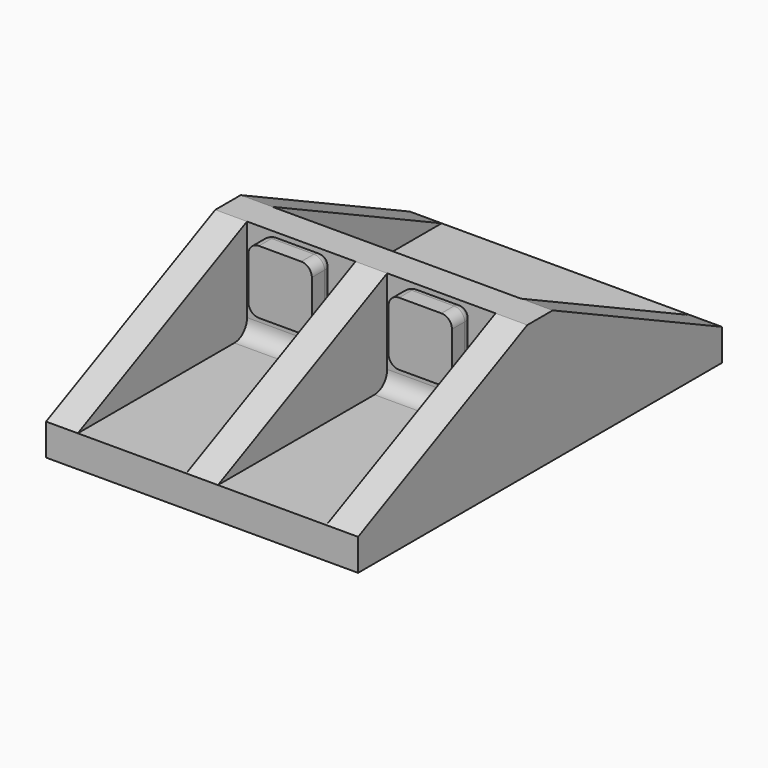
from build123d import *

# Parameters (mm, degrees)
F0_W             = 59
F0_H             = 86
F1_DEPTH         = 6
F3_DEPTH         = 19
F5_DEPTH         = 59.001
F7_R             = 3
F6_W             = 12
F6_H             = 12
F8_DEPTH         = 5
F9_R             = 2
F10_T1_DEPTH     = 8
F10_S5_W         = 2
F10_S5_H         = 2
F10_T6_DEPTH     = 2
F10_S11_W        = 2
F10_S11_H        = 2
F10_T12_DEPTH    = 2
F10_S17_W        = 2
F10_S17_H        = 2
F10_T18_DEPTH    = 2
F10_S23_W        = 2
F10_S23_H        = 2
F10_T24_DEPTH    = 2
F10_S1_T1_DEPTH  = 8
F10_S1_S5_W      = 2
F10_S1_S5_H      = 2
F10_S1_T6_DEPTH  = 2
F10_S1_S11_W     = 2
F10_S1_S11_H     = 2
F10_S1_T12_DEPTH = 2
F10_S1_S17_W     = 2
F10_S1_S17_H     = 2
F10_S1_T18_DEPTH = 2
F10_S1_S23_W     = 2
F10_S1_S23_H     = 2
F10_S1_T24_DEPTH = 2


# Not quite as in the source:
# - a fillet or chamfer that OpenCascade refuses, or shapes differently, is made with other operations: its cross-section is extruded or revolved along the edge and cut away or added


with BuildPart() as f1:
    # F0 (on Top) → F1 (new body)
    with BuildSketch(Plane.XY):
        Rectangle(F0_W, F0_H)
    extrude(amount=F1_DEPTH)

    # F2 (on face) → F3 (join)
    with BuildSketch(Plane.XY.offset(6)):
        Polygon((-23.5, 43), (-29.5, 43), (-29.5, -43), (-23.5, -43), (-23.5, -3), (-3, -3), (-3, -43), (3, -43), (3, -3), (23.5, -3), (23.5, -43), (29.5, -43), (29.5, 43), (23.5, 43), (23.5, 3), (-23.5, 3), align=None)
    extrude(amount=F3_DEPTH)

    # F4 (on face) → F5 (cut, through all)
    with BuildSketch(Plane.YZ.offset(29.5)):
        Polygon((-43, 25), (-43, 6), (-3, 25), align=None)
        Polygon((43, 25), (3, 25), (43, 6), align=None)
    extrude(amount=-F5_DEPTH, mode=Mode.SUBTRACT)

    # F7
    f7_edges = [f1.edges().sort_by_distance(p)[0] for p in [
        (-13.25, -3, 6),
        (13.25, -3, 6),
        (0, 3, 6),
    ]]
    fillet(f7_edges, radius=F7_R)


with BuildPart() as f8:
    # F6 (on face) → F8 (new body)
    with BuildSketch(Plane.XZ.offset(3)):
        with Locations((-13.25, 19)):
            Rectangle(F6_W, F6_H)
        with Locations((13.25, 19)):
            Rectangle(F6_W, F6_H)
    extrude(amount=F8_DEPTH)

    # F9
    f9_edges = [f8.edges().sort_by_distance(p)[0] for p in [
        (-7.25, -3, 19),
        (-13.25, -3, 25),
        (-19.25, -3, 19),
        (-13.25, -3, 13),
        (13.25, -3, 13),
        (7.25, -3, 19),
        (19.25, -3, 19),
        (13.25, -3, 25),
    ]]
    fillet(f9_edges, radius=F9_R)

    # F10: fillet of radius 2 on 4 edges, made by hand

    # F10_s2 → F10_t1 (cut)
    with BuildSketch(Plane.XZ.offset(5)):
        with BuildLine():
            ThreePointArc((-7.25, 15), (-7.8357864376, 13.5857864376), (-9.25, 13))
            Line((-9.25, 13), (-7.25, 13))
            Line((-7.25, 13), (-7.25, 15))
        make_face()
        with BuildLine():
            ThreePointArc((-19.25, 15), (-18.6642135624, 13.5857864376), (-17.25, 13))
            Line((-17.25, 13), (-19.25, 13))
            Line((-19.25, 13), (-19.25, 15))
        make_face()
        with BuildLine():
            ThreePointArc((-9.25, 25), (-7.8357864376, 24.4142135624), (-7.25, 23))
            Line((-7.25, 23), (-7.25, 25))
            Line((-7.25, 25), (-9.25, 25))
        make_face()
        with BuildLine():
            ThreePointArc((-17.25, 25), (-18.6642135624, 24.4142135624), (-19.25, 23))
            Line((-19.25, 23), (-19.25, 25))
            Line((-19.25, 25), (-17.25, 25))
        make_face()
    extrude(amount=F10_T1_DEPTH, mode=Mode.SUBTRACT)


with BuildPart() as f10_tool4:
    # F10_s5 → F10_t6 (new body)
    with BuildSketch(Plane.XY.offset(23)):
        with Locations((-18.25, -4)):
            Rectangle(F10_S5_W, F10_S5_H)
    extrude(amount=F10_T6_DEPTH)

    # F10_s7 → F10_t8 (revolve, cut)
    with BuildSketch(Plane(origin=(-17.25, -5, 23), x_dir=(0.7071067812, -0.7071067812, 0), z_dir=(-0.7071067812, -0.7071067812, 0))):
        with BuildLine():
            ThreePointArc((0, -2), (2, 0), (0, 2))
            Line((0, 2), (0, -2))
        make_face()
    revolve(axis=Axis((-17.25, -5, 23), (0, 0, 1)), mode=Mode.SUBTRACT)


with BuildPart() as f8_1:
    add(f8.part)

    # F10_t3: cut F10_tool4
    add(f10_tool4.part, mode=Mode.SUBTRACT)


with BuildPart() as f10_tool10:
    # F10_s11 → F10_t12 (new body)
    with BuildSketch(Plane.XY.offset(23)):
        with Locations((-8.25, -4)):
            Rectangle(F10_S11_W, F10_S11_H)
    extrude(amount=F10_T12_DEPTH)

    # F10_s13 → F10_t14 (revolve, cut)
    with BuildSketch(Plane(origin=(-9.25, -5, 23), x_dir=(-0.7071067812, -0.7071067812, 0), z_dir=(-0.7071067812, 0.7071067812, 0))):
        with BuildLine():
            ThreePointArc((0, -2), (2, 0), (0, 2))
            Line((0, 2), (0, -2))
        make_face()
    revolve(axis=Axis((-9.25, -5, 23), (0, 0, 1)), mode=Mode.SUBTRACT)


with BuildPart() as f8_2:
    add(f8_1.part)

    # F10_t9: cut F10_tool10
    add(f10_tool10.part, mode=Mode.SUBTRACT)


with BuildPart() as f10_tool16:
    # F10_s17 → F10_t18 (new body)
    with BuildSketch(Plane.YZ.offset(-17.25)):
        with Locations((-4, 14)):
            Rectangle(F10_S17_W, F10_S17_H)
    extrude(amount=-F10_T18_DEPTH)

    # F10_s19 → F10_t20 (revolve, cut)
    with BuildSketch(Plane(origin=(-17.25, -5, 15), x_dir=(0, -0.7071067812, 0.7071067812), z_dir=(0, -0.7071067812, -0.7071067812))):
        with BuildLine():
            ThreePointArc((0, -2), (2, 0), (0, 2))
            Line((0, 2), (0, -2))
        make_face()
    revolve(axis=Axis((-17.25, -5, 15), (-1, 0, 0)), mode=Mode.SUBTRACT)


with BuildPart() as f8_3:
    add(f8_2.part)

    # F10_t15: cut F10_tool16
    add(f10_tool16.part, mode=Mode.SUBTRACT)


with BuildPart() as f10_tool22:
    # F10_s23 → F10_t24 (new body)
    with BuildSketch(Plane.YZ.offset(-9.25)):
        with Locations((-4, 14)):
            Rectangle(F10_S23_W, F10_S23_H)
    extrude(amount=F10_T24_DEPTH)

    # F10_s25 → F10_t26 (revolve, cut)
    with BuildSketch(Plane(origin=(-9.25, -5, 15), x_dir=(0, -0.7071067812, 0.7071067812), z_dir=(0, 0.7071067812, 0.7071067812))):
        with BuildLine():
            ThreePointArc((0, -2), (2, 0), (0, 2))
            Line((0, 2), (0, -2))
        make_face()
    revolve(axis=Axis((-9.25, -5, 15), (1, 0, 0)), mode=Mode.SUBTRACT)


with BuildPart() as f8_4:
    add(f8_3.part)

    # F10_t21: cut F10_tool22
    add(f10_tool22.part, mode=Mode.SUBTRACT)

    # F10#s1: fillet of radius 2 on 4 edges, made by hand

    # F10_s1_s2 → F10_s1_t1 (cut)
    with BuildSketch(Plane.XZ.offset(5)):
        with BuildLine():
            ThreePointArc((19.25, 15), (18.6642135624, 13.5857864376), (17.25, 13))
            Line((17.25, 13), (19.25, 13))
            Line((19.25, 13), (19.25, 15))
        make_face()
        with BuildLine():
            ThreePointArc((17.25, 25), (18.6642135624, 24.4142135624), (19.25, 23))
            Line((19.25, 23), (19.25, 25))
            Line((19.25, 25), (17.25, 25))
        make_face()
        with BuildLine():
            ThreePointArc((7.25, 15), (7.8357864376, 13.5857864376), (9.25, 13))
            Line((9.25, 13), (7.25, 13))
            Line((7.25, 13), (7.25, 15))
        make_face()
        with BuildLine():
            ThreePointArc((9.25, 25), (7.8357864376, 24.4142135624), (7.25, 23))
            Line((7.25, 23), (7.25, 25))
            Line((7.25, 25), (9.25, 25))
        make_face()
    extrude(amount=F10_S1_T1_DEPTH, mode=Mode.SUBTRACT)


with BuildPart() as f10_s1_tool4:
    # F10_s1_s5 → F10_s1_t6 (new body)
    with BuildSketch(Plane.XY.offset(23)):
        with Locations((8.25, -4)):
            Rectangle(F10_S1_S5_W, F10_S1_S5_H)
    extrude(amount=F10_S1_T6_DEPTH)

    # F10_s1_s7 → F10_s1_t8 (revolve, cut)
    with BuildSketch(Plane(origin=(9.25, -5, 23), x_dir=(0.7071067812, -0.7071067812, 0), z_dir=(-0.7071067812, -0.7071067812, 0))):
        with BuildLine():
            ThreePointArc((0, -2), (2, 0), (0, 2))
            Line((0, 2), (0, -2))
        make_face()
    revolve(axis=Axis((9.25, -5, 23), (0, 0, 1)), mode=Mode.SUBTRACT)


with BuildPart() as f8_5:
    add(f8_4.part)

    # F10_s1_t3: cut F10_s1_tool4
    add(f10_s1_tool4.part, mode=Mode.SUBTRACT)


with BuildPart() as f10_s1_tool10:
    # F10_s1_s11 → F10_s1_t12 (new body)
    with BuildSketch(Plane.YZ.offset(9.25)):
        with Locations((-4, 14)):
            Rectangle(F10_S1_S11_W, F10_S1_S11_H)
    extrude(amount=-F10_S1_T12_DEPTH)

    # F10_s1_s13 → F10_s1_t14 (revolve, cut)
    with BuildSketch(Plane(origin=(9.25, -5, 15), x_dir=(0, -0.7071067812, 0.7071067812), z_dir=(0, -0.7071067812, -0.7071067812))):
        with BuildLine():
            ThreePointArc((0, -2), (2, 0), (0, 2))
            Line((0, 2), (0, -2))
        make_face()
    revolve(axis=Axis((9.25, -5, 15), (-1, 0, 0)), mode=Mode.SUBTRACT)


with BuildPart() as f8_6:
    add(f8_5.part)

    # F10_s1_t9: cut F10_s1_tool10
    add(f10_s1_tool10.part, mode=Mode.SUBTRACT)


with BuildPart() as f10_s1_tool16:
    # F10_s1_s17 → F10_s1_t18 (new body)
    with BuildSketch(Plane.XY.offset(23)):
        with Locations((18.25, -4)):
            Rectangle(F10_S1_S17_W, F10_S1_S17_H)
    extrude(amount=F10_S1_T18_DEPTH)

    # F10_s1_s19 → F10_s1_t20 (revolve, cut)
    with BuildSketch(Plane(origin=(17.25, -5, 23), x_dir=(-0.7071067812, -0.7071067812, 0), z_dir=(-0.7071067812, 0.7071067812, 0))):
        with BuildLine():
            ThreePointArc((0, -2), (2, 0), (0, 2))
            Line((0, 2), (0, -2))
        make_face()
    revolve(axis=Axis((17.25, -5, 23), (0, 0, 1)), mode=Mode.SUBTRACT)


with BuildPart() as f8_7:
    add(f8_6.part)

    # F10_s1_t15: cut F10_s1_tool16
    add(f10_s1_tool16.part, mode=Mode.SUBTRACT)


with BuildPart() as f10_s1_tool22:
    # F10_s1_s23 → F10_s1_t24 (new body)
    with BuildSketch(Plane.YZ.offset(17.25)):
        with Locations((-4, 14)):
            Rectangle(F10_S1_S23_W, F10_S1_S23_H)
    extrude(amount=F10_S1_T24_DEPTH)

    # F10_s1_s25 → F10_s1_t26 (revolve, cut)
    with BuildSketch(Plane(origin=(17.25, -5, 15), x_dir=(0, -0.7071067812, 0.7071067812), z_dir=(0, 0.7071067812, 0.7071067812))):
        with BuildLine():
            ThreePointArc((0, -2), (2, 0), (0, 2))
            Line((0, 2), (0, -2))
        make_face()
    revolve(axis=Axis((17.25, -5, 15), (1, 0, 0)), mode=Mode.SUBTRACT)


with BuildPart() as f8_8:
    add(f8_7.part)

    # F10_s1_t21: cut F10_s1_tool22
    add(f10_s1_tool22.part, mode=Mode.SUBTRACT)


solid = Compound([f1.part, f8_8.part])
